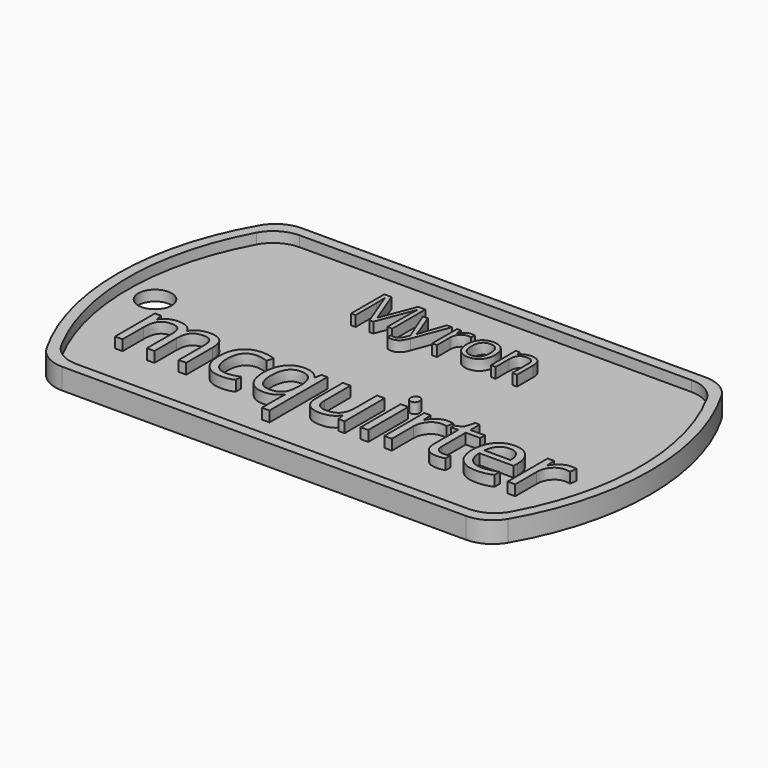
from build123d import *

# Parameters (mm, degrees)
F1_DEPTH     = 1
F3_DEPTH     = 1
F4_R         = 1.5875
F5_DEPTH     = 1
F6_TEXT_SIZE = 5.5389556806
F8_DEPTH     = 1
F7_TEXT_SIZE = 8.8912402538
F9_DEPTH     = 1


# Not quite as in the source:
# - Text() gives the source's letters only with a copy of the font that has no kerning and outlines rounded to 1/6400 em; it was checked with that copy


with BuildPart() as f1:
    # F0 (on Top) → F1 (new body)
    with BuildSketch(Plane.XY):
        with BuildLine():
            ThreePointArc((-19.2474145991, 14.2875), (-20.8349145991, 13.862130657), (-21.9970452561, 12.7))
            ThreePointArc((-21.9970452561, 12.7), (-25.4, 0), (-21.9970452561, -12.7))
            ThreePointArc((-21.9970452561, -12.7), (-20.8349145991, -13.862130657), (-19.2474145991, -14.2875))
            Line((-19.2474145991, -14.2875), (19.2474145991, -14.2875))
            ThreePointArc((19.2474145991, -14.2875), (20.8349145991, -13.862130657), (21.9970452561, -12.7))
            ThreePointArc((21.9970452561, -12.7), (25.4, 0), (21.9970452561, 12.7))
            ThreePointArc((21.9970452561, 12.7), (20.8349145991, 13.862130657), (19.2474145991, 14.2875))
            Line((19.2474145991, 14.2875), (-19.2474145991, 14.2875))
        make_face()
    extrude(amount=F1_DEPTH)

    # F2 (on face) → F3 (join)
    with BuildSketch(Plane.XY.offset(1)):
        with BuildLine():
            Line((19.2474145991, 14.2875), (-19.2474145991, 14.2875))
            ThreePointArc((-19.2474145991, 14.2875), (-20.8349145991, 13.862130657), (-21.9970452561, 12.7))
            ThreePointArc((-21.9970452561, 12.7), (-25.4, 0), (-21.9970452561, -12.7))
            ThreePointArc((-21.9970452561, -12.7), (-20.8349145991, -13.862130657), (-19.2474145991, -14.2875))
            Line((-19.2474145991, -14.2875), (19.2474145991, -14.2875))
            ThreePointArc((19.2474145991, -14.2875), (20.8349145991, -13.862130657), (21.9970452561, -12.7))
            ThreePointArc((21.9970452561, -12.7), (25.4, 0), (21.9970452561, 12.7))
            ThreePointArc((21.9970452561, 12.7), (20.8349145991, 13.862130657), (19.2474145991, 14.2875))
        make_face()
        with BuildLine():
            ThreePointArc((-21.4526124879, 11.6252061249), (-20.2856017842, 12.8404540819), (-18.6611352482, 13.2875))
            Line((-18.6611352482, 13.2875), (18.6611352482, 13.2875))
            ThreePointArc((18.6611352482, 13.2875), (20.2856017842, 12.8404540819), (21.4526124879, 11.6252061249))
            ThreePointArc((21.4526124879, 11.6252061249), (24.4, 0), (21.4526124879, -11.6252061249))
            ThreePointArc((21.4526124879, -11.6252061249), (20.2856017842, -12.8404540819), (18.6611352482, -13.2875))
            Line((18.6611352482, -13.2875), (-18.6611352482, -13.2875))
            ThreePointArc((-18.6611352482, -13.2875), (-20.2856017842, -12.8404540819), (-21.4526124879, -11.6252061249))
            ThreePointArc((-21.4526124879, -11.6252061249), (-24.4, 0), (-21.4526124879, 11.6252061249))
        make_face(mode=Mode.SUBTRACT)
    extrude(amount=F3_DEPTH)

    # F4 (on face) → F5 (cut)
    with BuildSketch(Plane.XY.offset(1)):
        with Locations((-21.821282804, 0)):
            Circle(F4_R)
    extrude(amount=-F5_DEPTH, mode=Mode.SUBTRACT)

    # F6 (on face) → F8 (join)
    with BuildSketch(Plane.XY.offset(1)):
        with Locations((-8.3560339213, 5.8458211432)):
            Text('Myron', F6_TEXT_SIZE, font='Open Sans', text_align=(TextAlign.LEFT, TextAlign.BOTTOM))
    extrude(amount=F8_DEPTH)

    # F7 (on face) → F9 (join)
    with BuildSketch(Plane.XY.offset(1)):
        with Locations((-19.9755819049, -8.0227273284)):
            Text('mcquirter', F7_TEXT_SIZE, font='Open Sans', text_align=(TextAlign.LEFT, TextAlign.BOTTOM))
    extrude(amount=F9_DEPTH)


solid = f1.part
